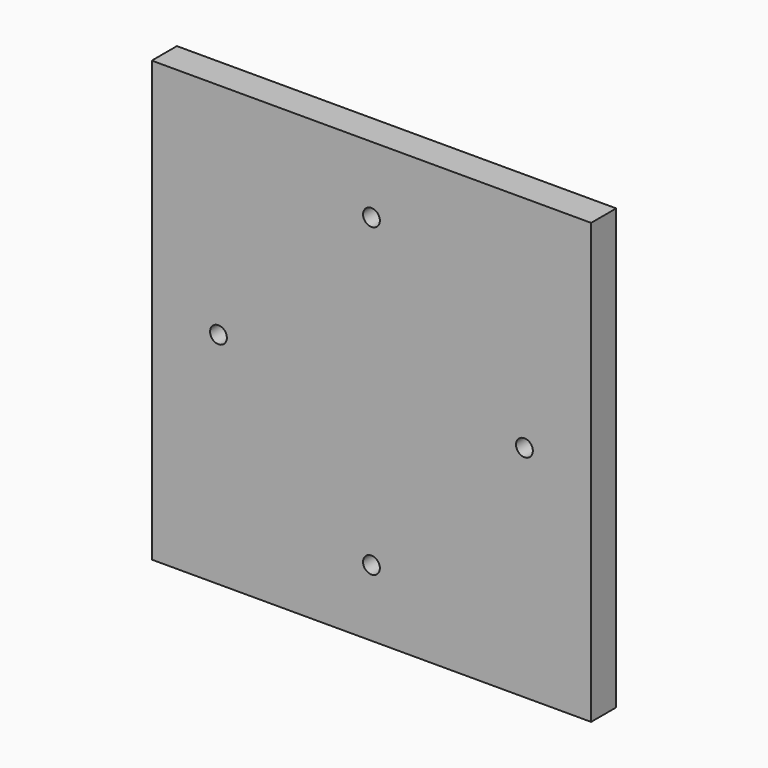
from build123d import *

# Parameters (mm, degrees)
F0_W     = 177.8
F0_H     = 177.8
F1_DEPTH = 12.7
F2_D     = 6.8


# Not quite as in the source:
# - a length typed as a fraction of an inch, garbled in the dataset ("3 / 203.2 mm" for 3/8 in), is restored


with BuildPart() as f1:
    # F0 (on Front) → F1 (new body)
    with BuildSketch(Plane.XZ):
        with Locations((0, -7.6e-09)):
            Rectangle(F0_W, F0_H)
    extrude(amount=F1_DEPTH)

    # F2 (through all)
    with Locations(Plane(origin=(0, 0, 0), x_dir=(1, 0, 0), z_dir=(0, 1, 0))):
        with Locations((-61.9125, 7.6e-09), (0, -61.9124999924), (61.9125, 7.6e-09), (0, 61.9124999319)):
            Hole(F2_D / 2)


solid = f1.part
